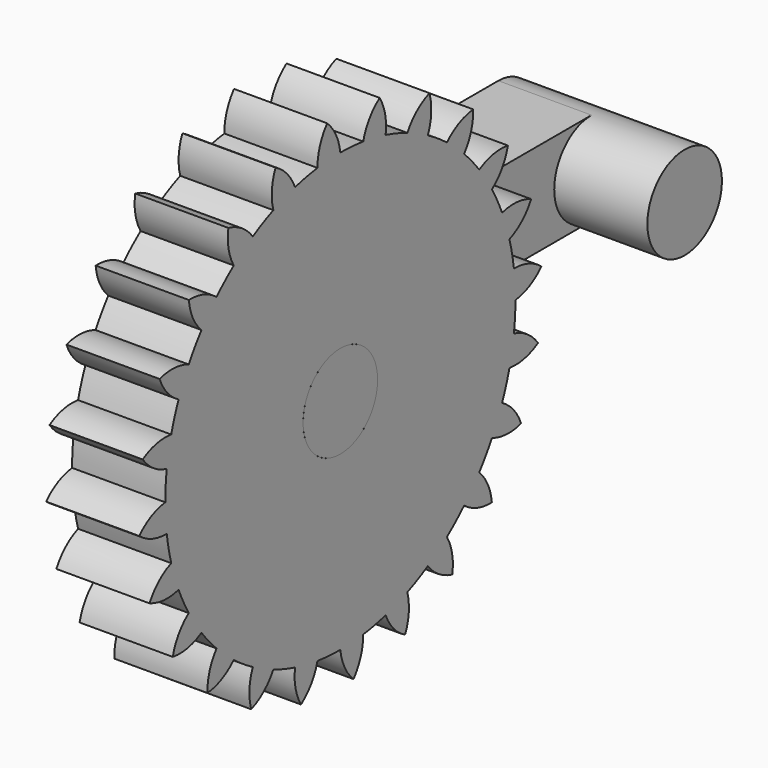
from build123d import *

# Parameters (mm, degrees)
F1_DEPTH = 25.4
F2_DEPTH = 50.8
F3_R     = 12.7
F4_DEPTH = 25.4
F5_COUNT = 24
F5_ANGLE = 345


with BuildPart() as f1:
    # F0 (on Right) → F1 (new body)
    with BuildSketch(Plane.YZ):
        with BuildLine():
            ThreePointArc((12.7, 12.7), (8.9802561211, 3.7197438789), (0, 0))
            Line((0, 0), (117.348, 0))
            ThreePointArc((117.348, 0), (104.648, 12.7), (117.348, 25.4))
            Line((117.348, 25.4), (0, 25.4))
            ThreePointArc((0, 25.4), (8.9802561211, 21.6802561211), (12.7, 12.7))
        make_face()
        with BuildLine():
            ThreePointArc((0, 25.4), (-12.7, 12.7), (0, 0))
            Line((0, 0), (0, 25.4))
        make_face()
        with BuildLine():
            Line((0, 25.4), (0, 0))
            ThreePointArc((0, 0), (8.9802561211, 3.7197438789), (12.7, 12.7))
            ThreePointArc((12.7, 12.7), (8.9802561211, 21.6802561211), (0, 25.4))
        make_face()
        with BuildLine():
            ThreePointArc((117.348, 25.4), (104.648, 12.7), (117.348, 0))
            Line((117.348, 0), (117.348, 25.4))
        make_face()
        with BuildLine():
            Line((117.348, 25.4), (117.348, 0))
            ThreePointArc((117.348, 0), (126.3282561211, 3.7197438789), (130.048, 12.7))
            ThreePointArc((130.048, 12.7), (126.3282561211, 21.6802561211), (117.348, 25.4))
        make_face()
    extrude(amount=F1_DEPTH)

    # F0 (on Right) → F2 (join)
    with BuildSketch(Plane.YZ):
        with BuildLine():
            ThreePointArc((0, 25.4), (-12.7, 12.7), (0, 0))
            Line((0, 0), (0, 25.4))
        make_face()
        with BuildLine():
            Line((0, 25.4), (0, 0))
            ThreePointArc((0, 0), (8.9802561211, 3.7197438789), (12.7, 12.7))
            ThreePointArc((12.7, 12.7), (8.9802561211, 21.6802561211), (0, 25.4))
        make_face()
        with BuildLine():
            Line((117.348, 25.4), (117.348, 0))
            ThreePointArc((117.348, 0), (126.3282561211, 3.7197438789), (130.048, 12.7))
            ThreePointArc((130.048, 12.7), (126.3282561211, 21.6802561211), (117.348, 25.4))
        make_face()
        with BuildLine():
            ThreePointArc((117.348, 25.4), (104.648, 12.7), (117.348, 0))
            Line((117.348, 0), (117.348, 25.4))
        make_face()
    extrude(amount=F2_DEPTH)


with BuildPart() as f4:
    # F3 (on face) → F4 (new body)
    with BuildSketch(Plane.YZ.offset(50.8)):
        with BuildLine():
            ThreePointArc((-7.7840813249, 71.8605817315), (-39.3451805995, -32.1611537578), (59.6704814199, 12.7))
            ThreePointArc((59.6704814199, 12.7), (42.1918046526, 54.8949993843), (-0.0045180328, 72.3704812489))
            ThreePointArc((-0.0045180328, 72.3704812489), (-3.9026362075, 72.2427223388), (-7.7840813249, 71.8605817315))
        make_face()
        with Locations((0, 12.7)):
            Circle(F3_R, mode=Mode.SUBTRACT)
        with BuildLine():
            ThreePointArc((-7.7840813249, 71.8605817315), (-3.9026362075, 72.2427223388), (-0.0045180328, 72.3704812489))
            ThreePointArc((-0.0045180328, 72.3704812489), (-1.463981414, 77.1998216133), (-4.492027974, 81.2351029848))
            ThreePointArc((-4.492027974, 81.2351029848), (-6.967459264, 76.8391046175), (-7.7840813249, 71.8605817315))
        make_face()
    extrude(amount=-F4_DEPTH)

    # F5: F4 ×24 about axis
    f5_axis = Axis((50.8, 0, 12.7), (1, 0, 0))


with BuildPart() as f4_1:
    add(f4.part)
    for i in range(1, F5_COUNT):
        add(f4.part.rotate(f5_axis, i * F5_ANGLE / (F5_COUNT - 1)))


solid = Compound([f1.part, f4_1.part])
